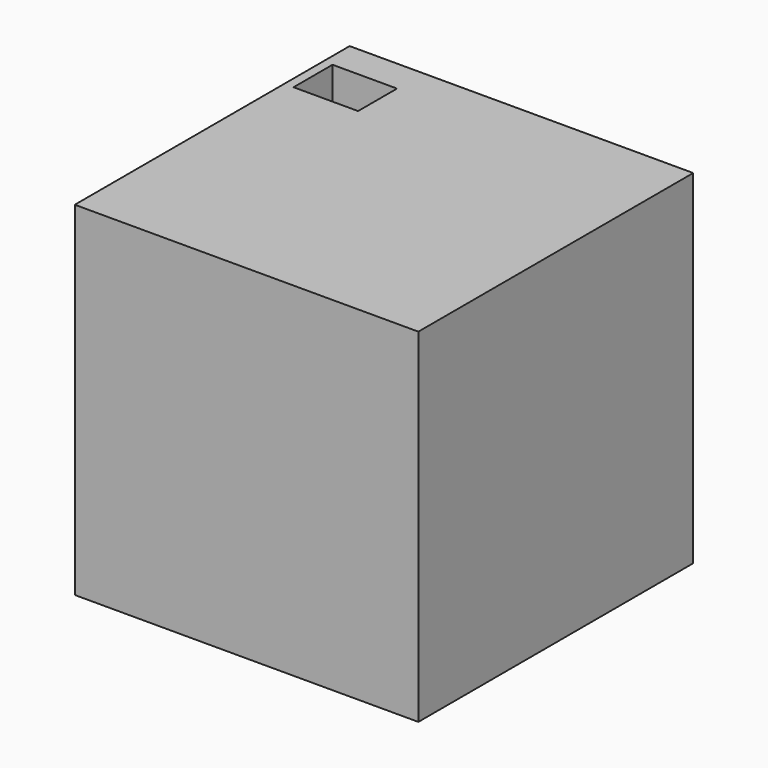
from build123d import *

# Parameters (mm, degrees)
F1_W       = 152.4
F1_H       = 152.4
F2_DEPTH   = 76.2
F3_W       = 28.6219716072
F3_H       = 21.6014906764
F2_FACE1_W = 152.4
F2_FACE1_H = 152.4
F4_DEPTH   = 81.28
F5_W       = 28.6219716072
F5_H       = 21.6014906764
F6_DEPTH   = 74.676
F7_W       = 7.5074806809
F7_H       = 1.7182230949
F7_W_2     = 6.0756318271
F7_H_2     = 1.7272
F8_DEPTH   = 40.64


# Not quite as in the source:
# - a variable given as a bare number and used for a length is read in inches; the dataset says mm whatever the document's units were


with BuildPart() as f2:
    # F1 (on Front) → F2 (new body, symmetric)
    with BuildSketch(Plane.XZ):
        Rectangle(F1_W, F1_H)
    extrude(amount=F2_DEPTH, both=True)

    # F3 (on face) + F2_face1 (on face) → F4 (cut)
    with BuildSketch(Plane.XY.offset(76.2)):
        with Locations((-57.7839799225, 50.7634989917)):
            Rectangle(F3_W, F3_H)
    with BuildSketch(Plane(origin=(0, 0, -76.2), x_dir=(1, 0, 0), z_dir=(0, 0, -1))):
        Rectangle(F2_FACE1_W, F2_FACE1_H)
    extrude(amount=-F4_DEPTH, dir=(0, 0, 1), mode=Mode.SUBTRACT)

    # F5 (on face) → F6 (join)
    with BuildSketch(Plane(origin=(0, 0, -76.2), x_dir=(1, 0, 0), z_dir=(0, 0, -1))):
        with Locations((-57.7839799225, -50.7634989917)):
            Rectangle(F5_W, F5_H)
    extrude(amount=F6_DEPTH)

    # F7 (on face) → F8 (join)
    with BuildSketch(Plane(origin=(-72.0949657261, 0, 0), x_dir=(0, -1, 0), z_dir=(-1, 0, 0))):
        with Locations((-57.8105039895, -147.6161032915)):
            Rectangle(F7_W, F7_H)
        with Locations((-43.0005695671, -147.3252443232)):
            Rectangle(F7_W_2, F7_H_2)
    extrude(amount=F8_DEPTH)


solid = f2.part
